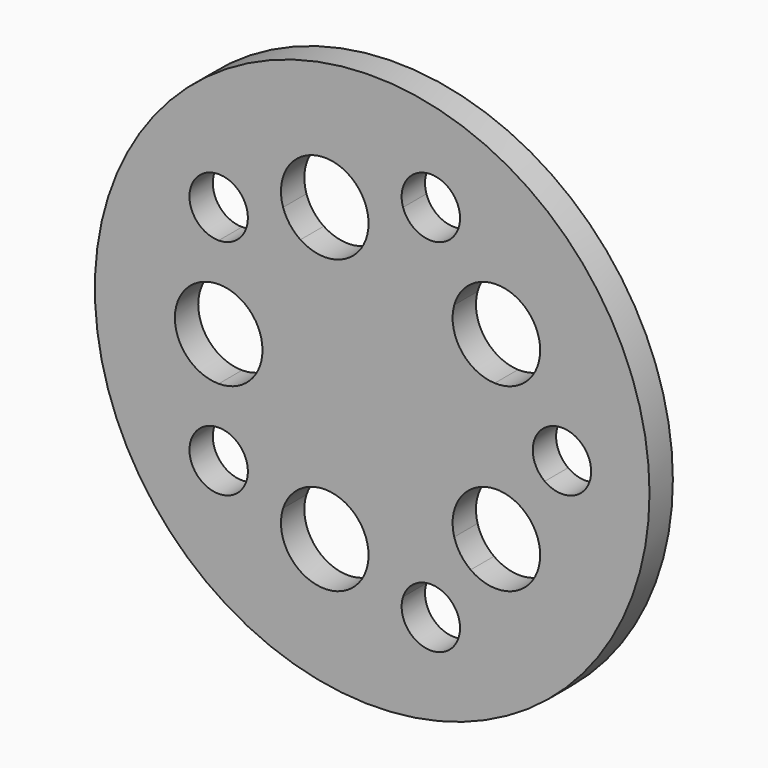
from build123d import *

# Parameters (mm, degrees)
F0_R     = 9.5
F1_DEPTH = 1


# Not quite as in the source:
# - a feature names something its author has since deleted; it is built from what else it names


with BuildPart() as f1:
    # F0 (on Front) → F1 (new body)
    with BuildSketch(Plane.XZ):
        Circle(F0_R)
        with BuildLine():
            Line((-6.1874431518, -2.6427799437), (-5.2586104634, -1.91030207))
            Line((-5.2586104634, -1.91030207), (-5.2586104634, -1.5))
            ThreePointArc((-5.2586104634, -1.5), (-6.7586104634, 0), (-5.2586104634, 1.5))
            Line((-5.2586104634, 1.5), (-5.2586104634, 1.91030207))
            Line((-5.2586104634, 1.91030207), (-6.1874431518, 2.6427799437))
            ThreePointArc((-6.1874431518, 2.6427799437), (-6.472135955, 4.7022820183), (-4.4254581722, 5.0679442137))
            Line((-4.4254581722, 5.0679442137), (-3.4418052317, 4.4109199439))
            Line((-3.4418052317, 4.4109199439), (-3.0515847744, 4.5377102563))
            ThreePointArc((-3.0515847744, 4.5377102563), (-2.0885254916, 6.4278205224), (-0.1984152256, 5.4647612395))
            Line((-0.1984152256, 5.4647612395), (0.1918052317, 5.5915515519))
            Line((0.1918052317, 5.5915515519), (0.601408001, 6.7012720437))
            ThreePointArc((0.601408001, 6.7012720437), (2.2724250824, 7.6584857382), (3.5086104634, 6.1818673559))
            ThreePointArc((3.5086104634, 6.1818673559), (3.4944811986, 5.976469794), (3.4523595855, 5.7749417209))
            Line((3.4523595855, 5.7749417209), (3.1314578476, 4.6364005169))
            Line((3.1314578476, 4.6364005169), (3.3726273533, 4.3044591695))
            ThreePointArc((3.3726273533, 4.3044591695), (4.9352909813, 4.4274434642), (5.7543052317, 3.090933678))
            ThreePointArc((5.7543052317, 3.090933678), (5.590815018, 2.4099479283), (5.1359831102, 1.8774081864))
            Line((5.1359831102, 1.8774081864), (5.3771526159, 1.545466839))
            Line((5.3771526159, 1.545466839), (6.5591337375, 1.4988339471))
            ThreePointArc((6.5591337375, 1.4988339471), (7.5813650184, 1.0395430231), (8, 0))
            ThreePointArc((8, 0), (7.5813650184, -1.0395430231), (6.5591337375, -1.4988339471))
            Line((6.5591337375, -1.4988339471), (5.3771526159, -1.545466839))
            Line((5.3771526159, -1.545466839), (5.1359831102, -1.8774081864))
            ThreePointArc((5.1359831102, -1.8774081864), (5.590815018, -2.4099479283), (5.7543052317, -3.090933678))
            ThreePointArc((5.7543052317, -3.090933678), (4.9352909813, -4.4274434642), (3.3726273533, -4.3044591695))
            Line((3.3726273533, -4.3044591695), (3.1314578476, -4.6364005169))
            Line((3.1314578476, -4.6364005169), (3.4523595855, -5.7749417209))
            ThreePointArc((3.4523595855, -5.7749417209), (3.4944811986, -5.976469794), (3.5086104634, -6.1818673559))
            ThreePointArc((3.5086104634, -6.1818673559), (2.2724250824, -7.6584857382), (0.601408001, -6.7012720437))
            Line((0.601408001, -6.7012720437), (0.1918052317, -5.5915515519))
            Line((0.1918052317, -5.5915515519), (-0.1984152256, -5.4647612395))
            ThreePointArc((-0.1984152256, -5.4647612395), (-2.0885254916, -6.4278205224), (-3.0515847744, -4.5377102563))
            Line((-3.0515847744, -4.5377102563), (-3.4418052317, -4.4109199439))
            Line((-3.4418052317, -4.4109199439), (-4.4254581722, -5.0679442137))
            ThreePointArc((-4.4254581722, -5.0679442137), (-6.472135955, -4.7022820183), (-6.1874431518, -2.6427799437))
        make_face(mode=Mode.SUBTRACT)
        with BuildLine():
            Line((-5.2586104634, -1.91030207), (-5.2586104634, -2.3206041399))
            ThreePointArc((-5.2586104634, -2.3206041399), (-4.1979502917, -2.7599439681), (-3.7586104634, -3.8206041399))
            ThreePointArc((-3.7586104634, -3.8206041399), (-3.7770779525, -4.0552558375), (-3.832025689, -4.2841296315))
            Line((-3.832025689, -4.2841296315), (-3.4418052317, -4.4109199439))
            Line((-3.4418052317, -4.4109199439), (-2.4581522912, -3.7538956741))
            ThreePointArc((-2.4581522912, -3.7538956741), (-1.1614745084, -3.5746509735), (-0.2177975376, -4.4818310601))
            Line((-0.2177975376, -4.4818310601), (0.1918052317, -5.5915515519))
            Line((0.1918052317, -5.5915515519), (0.582025689, -5.7183418644))
            ThreePointArc((0.582025689, -5.7183418644), (1.5450849719, -4.7552825815), (2.8902883419, -4.9683418644))
            Line((2.8902883419, -4.9683418644), (3.1314578476, -4.6364005169))
            Line((3.1314578476, -4.6364005169), (2.8105561096, -3.497859313))
            ThreePointArc((2.8105561096, -3.497859313), (3.0407797402, -2.2092557995), (4.1951714942, -1.5920997308))
            Line((4.1951714942, -1.5920997308), (5.3771526159, -1.545466839))
            Line((5.3771526159, -1.545466839), (5.6183221216, -1.2135254916))
            ThreePointArc((5.6183221216, -1.2135254916), (5, 0), (5.6183221216, 1.2135254916))
            Line((5.6183221216, 1.2135254916), (5.3771526159, 1.545466839))
            Line((5.3771526159, 1.545466839), (4.1951714942, 1.5920997308))
            ThreePointArc((4.1951714942, 1.5920997308), (3.0407797402, 2.2092557995), (2.8105561096, 3.497859313))
            Line((2.8105561096, 3.497859313), (3.1314578476, 4.6364005169))
            Line((3.1314578476, 4.6364005169), (2.8902883419, 4.9683418644))
            ThreePointArc((2.8902883419, 4.9683418644), (1.5450849719, 4.7552825815), (0.582025689, 5.7183418644))
            Line((0.582025689, 5.7183418644), (0.1918052317, 5.5915515519))
            Line((0.1918052317, 5.5915515519), (-0.2177975376, 4.4818310601))
            ThreePointArc((-0.2177975376, 4.4818310601), (-1.1614745084, 3.5746509735), (-2.4581522912, 3.7538956741))
            Line((-2.4581522912, 3.7538956741), (-3.4418052317, 4.4109199439))
            Line((-3.4418052317, 4.4109199439), (-3.832025689, 4.2841296315))
            ThreePointArc((-3.832025689, 4.2841296315), (-3.7770779525, 4.0552558375), (-3.7586104634, 3.8206041399))
            ThreePointArc((-3.7586104634, 3.8206041399), (-4.1979502917, 2.7599439681), (-5.2586104634, 2.3206041399))
            Line((-5.2586104634, 2.3206041399), (-5.2586104634, 1.91030207))
            Line((-5.2586104634, 1.91030207), (-4.3297777751, 1.1778241962))
            ThreePointArc((-4.3297777751, 1.1778241962), (-3.9089347556, 0.6545039983), (-3.7586104634, 0))
            ThreePointArc((-3.7586104634, 0), (-3.9089347556, -0.6545039983), (-4.3297777751, -1.1778241962))
            Line((-4.3297777751, -1.1778241962), (-5.2586104634, -1.91030207))
        make_face()
        with BuildLine():
            ThreePointArc((1.5, 2), (2.2360679775, 1.1180339887), (2.5, 0))
            ThreePointArc((2.5, 0), (2.2360679775, -1.1180339887), (1.5, -2))
            ThreePointArc((1.5, -2), (-2.5, 0), (1.5, 2))
        make_face(mode=Mode.SUBTRACT)
        with BuildLine():
            Line((1.5, -2), (1.5, 2))
            ThreePointArc((1.5, 2), (-2.5, 0), (1.5, -2))
        make_face()
        with BuildLine():
            ThreePointArc((1.5, -2), (2.2360679775, -1.1180339887), (2.5, 0))
            ThreePointArc((2.5, 0), (2.2360679775, 1.1180339887), (1.5, 2))
            Line((1.5, 2), (1.5, -2))
        make_face()
        with BuildLine():
            ThreePointArc((-4.3075539471, -4.1296211343), (-6.0676274578, -4.4083893922), (-5.2586104634, -2.8206041399))
            Line((-5.2586104634, -2.8206041399), (-5.2586104634, -2.3206041399))
            ThreePointArc((-5.2586104634, -2.3206041399), (-5.7501710933, -2.403435079), (-6.1874431518, -2.6427799437))
            ThreePointArc((-6.1874431518, -2.6427799437), (-6.472135955, -4.7022820183), (-4.4254581722, -5.0679442137))
            ThreePointArc((-4.4254581722, -5.0679442137), (-4.0627031818, -4.7260354038), (-3.832025689, -4.2841296315))
            Line((-3.832025689, -4.2841296315), (-4.3075539471, -4.1296211343))
        make_face()
        with BuildLine():
            ThreePointArc((-6.1874431518, 2.6427799437), (-5.7501710933, 2.403435079), (-5.2586104634, 2.3206041399))
            Line((-5.2586104634, 2.3206041399), (-5.2586104634, 2.8206041399))
            ThreePointArc((-5.2586104634, 2.8206041399), (-6.0676274578, 4.4083893922), (-4.3075539471, 4.1296211343))
            Line((-4.3075539471, 4.1296211343), (-3.832025689, 4.2841296315))
            ThreePointArc((-3.832025689, 4.2841296315), (-4.0627031818, 4.7260354038), (-4.4254581722, 5.0679442137))
            ThreePointArc((-4.4254581722, 5.0679442137), (-6.472135955, 4.7022820183), (-6.1874431518, 2.6427799437))
        make_face()
        with BuildLine():
            Line((1.0575539471, -5.8728503615), (0.582025689, -5.7183418644))
            ThreePointArc((0.582025689, -5.7183418644), (0.508902005, -6.2114399724), (0.601408001, -6.7012720437))
            ThreePointArc((0.601408001, -6.7012720437), (2.2724250824, -7.6584857382), (3.5086104634, -6.1818673559))
            ThreePointArc((3.5086104634, -6.1818673559), (3.4944811986, -5.976469794), (3.4523595855, -5.7749417209))
            ThreePointArc((3.4523595855, -5.7749417209), (3.2392824408, -5.3242855906), (2.8902883419, -4.9683418644))
            Line((2.8902883419, -4.9683418644), (2.5963957157, -5.3728503615))
            ThreePointArc((2.5963957157, -5.3728503615), (2.8996169876, -5.7278768562), (3.0086104634, -6.1818673559))
            ThreePointArc((3.0086104634, -6.1818673559), (1.8521759984, -7.1695556965), (1.0575539471, -5.8728503615))
        make_face()
        with BuildLine():
            ThreePointArc((0.601408001, 6.7012720437), (0.508902005, 6.2114399724), (0.582025689, 5.7183418644))
            Line((0.582025689, 5.7183418644), (1.0575539471, 5.8728503615))
            ThreePointArc((1.0575539471, 5.8728503615), (1.8521759984, 7.1695556965), (3.0086104634, 6.1818673559))
            ThreePointArc((3.0086104634, 6.1818673559), (2.8996169876, 5.7278768562), (2.5963957157, 5.3728503615))
            Line((2.5963957157, 5.3728503615), (2.8902883419, 4.9683418644))
            ThreePointArc((2.8902883419, 4.9683418644), (3.2392824408, 5.3242855906), (3.4523595855, 5.7749417209))
            ThreePointArc((3.4523595855, 5.7749417209), (3.4944811986, 5.976469794), (3.5086104634, 6.1818673559))
            ThreePointArc((3.5086104634, 6.1818673559), (2.2724250824, 7.6584857382), (0.601408001, 6.7012720437))
        make_face()
        with BuildLine():
            Line((5.9122147477, -0.8090169944), (5.6183221216, -1.2135254916))
            ThreePointArc((5.6183221216, -1.2135254916), (6.0646898294, -1.435445943), (6.5591337375, -1.4988339471))
            ThreePointArc((6.5591337375, -1.4988339471), (7.5813650184, -1.0395430231), (8, 0))
            ThreePointArc((8, 0), (7.5813650184, 1.0395430231), (6.5591337375, 1.4988339471))
            ThreePointArc((6.5591337375, 1.4988339471), (6.0646898294, 1.435445943), (5.6183221216, 1.2135254916))
            Line((5.6183221216, 1.2135254916), (5.9122147477, 0.8090169944))
            ThreePointArc((5.9122147477, 0.8090169944), (6.9539904997, 0.8910065242), (7.5, 0))
            ThreePointArc((7.5, 0), (6.9539904997, -0.8910065242), (5.9122147477, -0.8090169944))
        make_face()
        with BuildLine():
            Line((-5.2586104634, -2.3206041399), (-5.2586104634, -2.8206041399))
            ThreePointArc((-5.2586104634, -2.8206041399), (-4.5515036823, -3.1134973587), (-4.2586104634, -3.8206041399))
            ThreePointArc((-4.2586104634, -3.8206041399), (-4.2709221228, -3.9770386049), (-4.3075539471, -4.1296211343))
            Line((-4.3075539471, -4.1296211343), (-3.832025689, -4.2841296315))
            ThreePointArc((-3.832025689, -4.2841296315), (-3.7770779525, -4.0552558375), (-3.7586104634, -3.8206041399))
            ThreePointArc((-3.7586104634, -3.8206041399), (-4.1979502917, -2.7599439681), (-5.2586104634, -2.3206041399))
        make_face()
        with BuildLine():
            Line((-5.2586104634, 2.8206041399), (-5.2586104634, 2.3206041399))
            ThreePointArc((-5.2586104634, 2.3206041399), (-4.1979502917, 2.7599439681), (-3.7586104634, 3.8206041399))
            ThreePointArc((-3.7586104634, 3.8206041399), (-3.7770779525, 4.0552558375), (-3.832025689, 4.2841296315))
            Line((-3.832025689, 4.2841296315), (-4.3075539471, 4.1296211343))
            ThreePointArc((-4.3075539471, 4.1296211343), (-4.2709221228, 3.9770386049), (-4.2586104634, 3.8206041399))
            ThreePointArc((-4.2586104634, 3.8206041399), (-4.5515036823, 3.1134973587), (-5.2586104634, 2.8206041399))
        make_face()
        with BuildLine():
            ThreePointArc((2.8902883419, -4.9683418644), (1.5450849719, -4.7552825815), (0.582025689, -5.7183418644))
            Line((0.582025689, -5.7183418644), (1.0575539471, -5.8728503615))
            ThreePointArc((1.0575539471, -5.8728503615), (1.6995934691, -5.2308108396), (2.5963957157, -5.3728503615))
            Line((2.5963957157, -5.3728503615), (2.8902883419, -4.9683418644))
        make_face()
        with BuildLine():
            Line((1.0575539471, 5.8728503615), (0.582025689, 5.7183418644))
            ThreePointArc((0.582025689, 5.7183418644), (1.5450849719, 4.7552825815), (2.8902883419, 4.9683418644))
            Line((2.8902883419, 4.9683418644), (2.5963957157, 5.3728503615))
            ThreePointArc((2.5963957157, 5.3728503615), (1.6995934691, 5.2308108396), (1.0575539471, 5.8728503615))
        make_face()
        with BuildLine():
            ThreePointArc((5.6183221216, 1.2135254916), (5, 0), (5.6183221216, -1.2135254916))
            Line((5.6183221216, -1.2135254916), (5.9122147477, -0.8090169944))
            ThreePointArc((5.9122147477, -0.8090169944), (5.5, 0), (5.9122147477, 0.8090169944))
            Line((5.9122147477, 0.8090169944), (5.6183221216, 1.2135254916))
        make_face()
        with BuildLine():
            ThreePointArc((-6.1874431518, -2.6427799437), (-5.7501710933, -2.403435079), (-5.2586104634, -2.3206041399))
            Line((-5.2586104634, -2.3206041399), (-5.2586104634, -1.91030207))
            Line((-5.2586104634, -1.91030207), (-6.1874431518, -2.6427799437))
        make_face()
        with BuildLine():
            Line((-3.4418052317, -4.4109199439), (-3.832025689, -4.2841296315))
            ThreePointArc((-3.832025689, -4.2841296315), (-4.0627031818, -4.7260354038), (-4.4254581722, -5.0679442137))
            Line((-4.4254581722, -5.0679442137), (-3.4418052317, -4.4109199439))
        make_face()
        with BuildLine():
            Line((-5.2586104634, -1.5), (-5.2586104634, -1.91030207))
            Line((-5.2586104634, -1.91030207), (-4.3297777751, -1.1778241962))
            ThreePointArc((-4.3297777751, -1.1778241962), (-4.7670498335, -1.4171690609), (-5.2586104634, -1.5))
        make_face()
        with BuildLine():
            Line((-2.4581522912, -3.7538956741), (-3.4418052317, -4.4109199439))
            Line((-3.4418052317, -4.4109199439), (-3.0515847744, -4.5377102563))
            ThreePointArc((-3.0515847744, -4.5377102563), (-2.8209072816, -4.095804484), (-2.4581522912, -3.7538956741))
        make_face()
        with BuildLine():
            Line((-5.2586104634, 1.91030207), (-5.2586104634, 1.5))
            ThreePointArc((-5.2586104634, 1.5), (-4.7670498335, 1.4171690609), (-4.3297777751, 1.1778241962))
            Line((-4.3297777751, 1.1778241962), (-5.2586104634, 1.91030207))
        make_face()
        with BuildLine():
            ThreePointArc((-0.125, -5.0012357479), (-0.1434674891, -5.2358874455), (-0.1984152256, -5.4647612395))
            Line((-0.1984152256, -5.4647612395), (0.1918052317, -5.5915515519))
            Line((0.1918052317, -5.5915515519), (-0.2177975376, -4.4818310601))
            ThreePointArc((-0.2177975376, -4.4818310601), (-0.1483816177, -4.737421129), (-0.125, -5.0012357479))
        make_face()
        with BuildLine():
            Line((-6.1874431518, 2.6427799437), (-5.2586104634, 1.91030207))
            Line((-5.2586104634, 1.91030207), (-5.2586104634, 2.3206041399))
            ThreePointArc((-5.2586104634, 2.3206041399), (-5.7501710933, 2.403435079), (-6.1874431518, 2.6427799437))
        make_face()
        with BuildLine():
            Line((0.582025689, -5.7183418644), (0.1918052317, -5.5915515519))
            Line((0.1918052317, -5.5915515519), (0.601408001, -6.7012720437))
            ThreePointArc((0.601408001, -6.7012720437), (0.508902005, -6.2114399724), (0.582025689, -5.7183418644))
        make_face()
        with BuildLine():
            Line((-3.4418052317, 4.4109199439), (-4.4254581722, 5.0679442137))
            ThreePointArc((-4.4254581722, 5.0679442137), (-4.0627031818, 4.7260354038), (-3.832025689, 4.2841296315))
            Line((-3.832025689, 4.2841296315), (-3.4418052317, 4.4109199439))
        make_face()
        with BuildLine():
            Line((3.1314578476, -4.6364005169), (2.8902883419, -4.9683418644))
            ThreePointArc((2.8902883419, -4.9683418644), (3.2392824408, -5.3242855906), (3.4523595855, -5.7749417209))
            Line((3.4523595855, -5.7749417209), (3.1314578476, -4.6364005169))
        make_face()
        with BuildLine():
            Line((-3.0515847744, 4.5377102563), (-3.4418052317, 4.4109199439))
            Line((-3.4418052317, 4.4109199439), (-2.4581522912, 3.7538956741))
            ThreePointArc((-2.4581522912, 3.7538956741), (-2.8209072816, 4.095804484), (-3.0515847744, 4.5377102563))
        make_face()
        with BuildLine():
            Line((2.8105561096, -3.497859313), (3.1314578476, -4.6364005169))
            Line((3.1314578476, -4.6364005169), (3.3726273533, -4.3044591695))
            ThreePointArc((3.3726273533, -4.3044591695), (3.0236332544, -3.9485154433), (2.8105561096, -3.497859313))
        make_face()
        with BuildLine():
            Line((0.1918052317, 5.5915515519), (-0.1984152256, 5.4647612395))
            ThreePointArc((-0.1984152256, 5.4647612395), (-0.1434674891, 5.2358874455), (-0.125, 5.0012357479))
            ThreePointArc((-0.125, 5.0012357479), (-0.1483816177, 4.737421129), (-0.2177975376, 4.4818310601))
            Line((-0.2177975376, 4.4818310601), (0.1918052317, 5.5915515519))
        make_face()
        with BuildLine():
            ThreePointArc((4.1951714942, -1.5920997308), (4.6896154024, -1.6554877349), (5.1359831102, -1.8774081864))
            Line((5.1359831102, -1.8774081864), (5.3771526159, -1.545466839))
            Line((5.3771526159, -1.545466839), (4.1951714942, -1.5920997308))
        make_face()
        with BuildLine():
            Line((0.601408001, 6.7012720437), (0.1918052317, 5.5915515519))
            Line((0.1918052317, 5.5915515519), (0.582025689, 5.7183418644))
            ThreePointArc((0.582025689, 5.7183418644), (0.508902005, 6.2114399724), (0.601408001, 6.7012720437))
        make_face()
        with BuildLine():
            Line((5.6183221216, -1.2135254916), (5.3771526159, -1.545466839))
            Line((5.3771526159, -1.545466839), (6.5591337375, -1.4988339471))
            ThreePointArc((6.5591337375, -1.4988339471), (6.0646898294, -1.435445943), (5.6183221216, -1.2135254916))
        make_face()
        with BuildLine():
            ThreePointArc((3.4523595855, 5.7749417209), (3.2392824408, 5.3242855906), (2.8902883419, 4.9683418644))
            Line((2.8902883419, 4.9683418644), (3.1314578476, 4.6364005169))
            Line((3.1314578476, 4.6364005169), (3.4523595855, 5.7749417209))
        make_face()
        with BuildLine():
            Line((5.3771526159, 1.545466839), (5.6183221216, 1.2135254916))
            ThreePointArc((5.6183221216, 1.2135254916), (6.0646898294, 1.435445943), (6.5591337375, 1.4988339471))
            Line((6.5591337375, 1.4988339471), (5.3771526159, 1.545466839))
        make_face()
        with BuildLine():
            Line((3.3726273533, 4.3044591695), (3.1314578476, 4.6364005169))
            Line((3.1314578476, 4.6364005169), (2.8105561096, 3.497859313))
            ThreePointArc((2.8105561096, 3.497859313), (3.0236332544, 3.9485154433), (3.3726273533, 4.3044591695))
        make_face()
        with BuildLine():
            Line((4.1951714942, 1.5920997308), (5.3771526159, 1.545466839))
            Line((5.3771526159, 1.545466839), (5.1359831102, 1.8774081864))
            ThreePointArc((5.1359831102, 1.8774081864), (4.6896154024, 1.6554877349), (4.1951714942, 1.5920997308))
        make_face()
    extrude(amount=F1_DEPTH)


solid = f1.part
